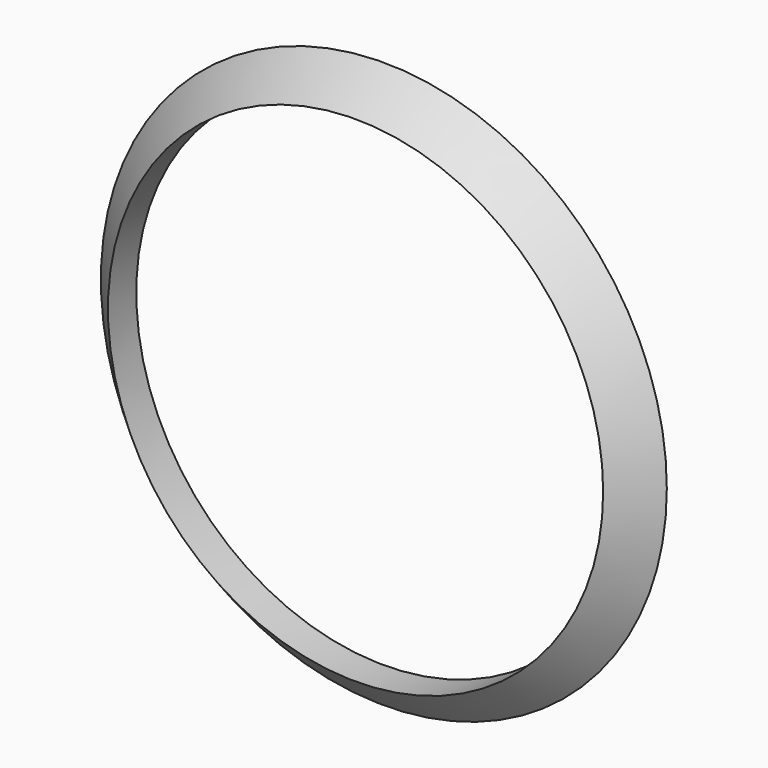
from build123d import *

# Parameters (mm, degrees)
F0_R     = 50.8
F0_R_2   = 44.45
F1_DEPTH = 6.35
F2_SIZE  = 6.34999


# Not quite as in the source:
# - a fillet or chamfer is up to 0.001 mm smaller than in the source, because OpenCascade refuses the exact size


with BuildPart() as f1:
    # F0 (on Front) → F1 (new body)
    with BuildSketch(Plane.XZ):
        Circle(F0_R)
        Circle(F0_R_2, mode=Mode.SUBTRACT)
    extrude(amount=F1_DEPTH)

    # F2 (size 6.35 in the source; OpenCascade refuses exactly that, so slightly less here)
    f2_edges = [f1.edges().sort_by_distance(p)[0] for p in [
        (-50.8, -6.35, 0),
    ]]
    chamfer(f2_edges, length=F2_SIZE)


solid = f1.part
